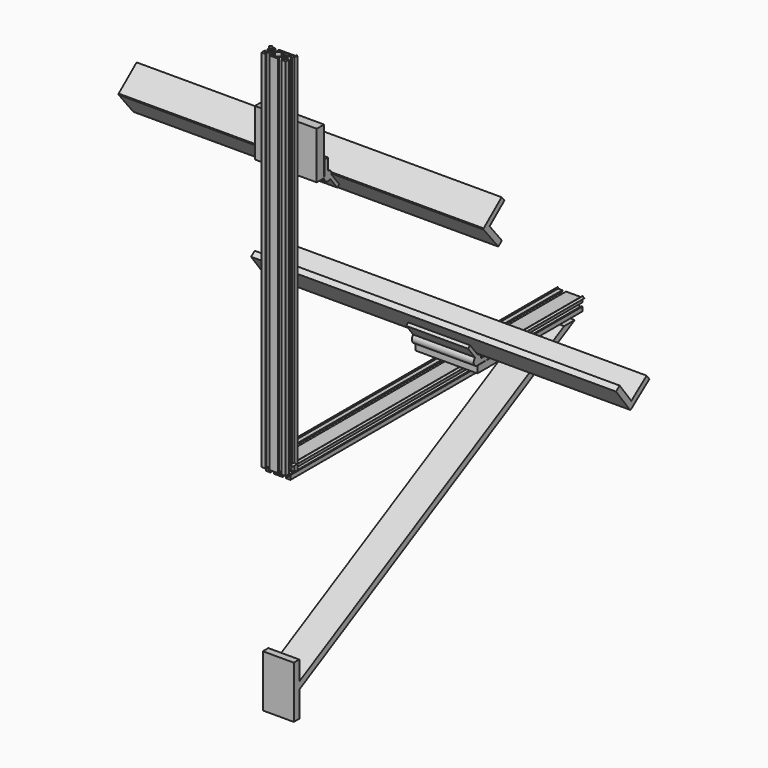
from build123d import *

# Parameters (mm, degrees)
F0_R          = 2.1
F1_DEPTH      = 600
F2_R          = 2.1
F3_DEPTH      = 600
F5_DEPTH      = 25.4
F5_DEPTH_BACK = 25.4
F6_W          = 67.6259994507
F6_H          = 11.4020574838
F7_DEPTH      = 50.8
F7_DEPTH_BACK = 50.8
F6_W_2        = 15.0790625318
F6_H_2        = 77.6842328595
F9_DEPTH      = 300
F9_DEPTH_BACK = 300


with BuildPart() as f1:
    # F0 (on Front) → F1 (new body)
    with BuildSketch(Plane.XZ):
        Polygon((16, -10), (20, -10), (20, -6), (20, -3), (18, -3), (18, -6), (17, -6), (13, -2), (13, 2), (17, 6), (18, 6), (18, 3), (20, 3), (20, 6), (20, 7.62), (20.4436164349, 7.62), (23.18, 10), (20.4436164349, 12.38), (20, 12.38), (20, 10), (16, 10), (-7, 10), (-7, 8), (-3, 8), (-8, 3), (-12, 3), (-16, 7), (-16, 8), (-13, 8), (-13, 10), (-16, 10), (-19, 10), (-20, 10), (-20, 12.38), (-20.4436164349, 12.38), (-23.18, 10), (-20.4436164349, 7.62), (-20, 7.62), (-20, 6), (-20, 3), (-18, 3), (-18, 6), (-17, 6), (-13, 2), (-13, -2), (-17, -6), (-18, -6), (-18, -3), (-20, -3), (-20, -6), (-20, -10), (-16, -10), (-13, -10), (-13, -8), (-16, -8), (-16, -7), (-12, -3), (-8, -3), (-3, -8), (-7, -8), (-7, -10), (-1, -10), (0, -10), (7, -10), (7, -8), (3, -8), (8, -3), (12, -3), (16, -7), (16, -8), (13, -8), (13, -10), align=None)
        with Locations((-10, 0)):
            Circle(F0_R, mode=Mode.SUBTRACT)
        Polygon((-2, -7), (-7, -2), (-7, 2), (-2, 7), (-1, 8), (1, 8), (2, 7), (7, 2), (7, -2), (2, -7), (1, -8), (-1, -8), align=None, mode=Mode.SUBTRACT)
        with Locations((10, 0)):
            Circle(F0_R, mode=Mode.SUBTRACT)
        Polygon((12, 3), (8, 3), (3, 8), (16, 8), (16, 7), align=None, mode=Mode.SUBTRACT)
    extrude(amount=-F1_DEPTH)

    # F2 (on Top) → F3 (join)
    with BuildSketch(Plane.XY):
        Polygon((16.4503816794, -10.3344274809), (20.4503816794, -10.3344274809), (20.4503816794, -6.3344274809), (20.4503816794, -3.3344274809), (18.4503816794, -3.3344274809), (18.4503816794, -6.3344274809), (17.4503816794, -6.3344274809), (13.4503816794, -2.3344274809), (13.4503816794, 1.6655725191), (17.4503816794, 5.6655725191), (18.4503816794, 5.6655725191), (18.4503816794, 2.6655725191), (20.4503816794, 2.6655725191), (20.4503816794, 5.6655725191), (20.4503816794, 7.2855725191), (20.8939981143, 7.2855725191), (23.6303816794, 9.6655725191), (20.8939981143, 12.0455725191), (20.4503816794, 12.0455725191), (20.4503816794, 9.6655725191), (16.4503816794, 9.6655725191), (-6.5496183206, 9.6655725191), (-6.5496183206, 7.6655725191), (-2.5496183206, 7.6655725191), (-7.5496183206, 2.6655725191), (-11.5496183206, 2.6655725191), (-15.5496183206, 6.6655725191), (-15.5496183206, 7.6655725191), (-12.5496183206, 7.6655725191), (-12.5496183206, 9.6655725191), (-15.5496183206, 9.6655725191), (-18.5496183206, 9.6655725191), (-19.5496183206, 9.6655725191), (-19.5496183206, 12.0455725191), (-19.9932347555, 12.0455725191), (-22.7296183206, 9.6655725191), (-19.9932347555, 7.2855725191), (-19.5496183206, 7.2855725191), (-19.5496183206, 5.6655725191), (-19.5496183206, 2.6655725191), (-17.5496183206, 2.6655725191), (-17.5496183206, 5.6655725191), (-16.5496183206, 5.6655725191), (-12.5496183206, 1.6655725191), (-12.5496183206, -2.3344274809), (-16.5496183206, -6.3344274809), (-17.5496183206, -6.3344274809), (-17.5496183206, -3.3344274809), (-19.5496183206, -3.3344274809), (-19.5496183206, -6.3344274809), (-19.5496183206, -10.3344274809), (-15.5496183206, -10.3344274809), (-12.5496183206, -10.3344274809), (-12.5496183206, -8.3344274809), (-15.5496183206, -8.3344274809), (-15.5496183206, -7.3344274809), (-11.5496183206, -3.3344274809), (-7.5496183206, -3.3344274809), (-2.5496183206, -8.3344274809), (-6.5496183206, -8.3344274809), (-6.5496183206, -10.3344274809), (-0.5496183206, -10.3344274809), (0.4503816794, -10.3344274809), (7.4503816794, -10.3344274809), (7.4503816794, -8.3344274809), (3.4503816794, -8.3344274809), (8.4503816794, -3.3344274809), (12.4503816794, -3.3344274809), (16.4503816794, -7.3344274809), (16.4503816794, -8.3344274809), (13.4503816794, -8.3344274809), (13.4503816794, -10.3344274809), align=None)
        with Locations((-9.5496183206, -0.3344274809)):
            Circle(F2_R, mode=Mode.SUBTRACT)
        Polygon((-1.5496183206, -7.3344274809), (-6.5496183206, -2.3344274809), (-6.5496183206, 1.6655725191), (-1.5496183206, 6.6655725191), (-0.5496183206, 7.6655725191), (1.4503816794, 7.6655725191), (2.4503816794, 6.6655725191), (7.4503816794, 1.6655725191), (7.4503816794, -2.3344274809), (2.4503816794, -7.3344274809), (1.4503816794, -8.3344274809), (-0.5496183206, -8.3344274809), align=None, mode=Mode.SUBTRACT)
        with Locations((10.4503816794, -0.3344274809)):
            Circle(F2_R, mode=Mode.SUBTRACT)
        Polygon((12.4503816794, 2.6655725191), (8.4503816794, 2.6655725191), (3.4503816794, 7.6655725191), (16.4503816794, 7.6655725191), (16.4503816794, 6.6655725191), align=None, mode=Mode.SUBTRACT)
    extrude(amount=F3_DEPTH)


with BuildPart() as f5:
    # F4 (on Right) → F5 (new body, two sides)
    with BuildSketch(Plane.YZ) as f5_sk:
        Polygon((577.4232465298, -11.5676193306), (577.0964622498, -11.5676193306), (577.0964622498, -11.7435521713), align=None)
        Polygon((577.0964622498, -11.7435521713), (577.0964622498, -11.5676193306), (555.6103307278, -11.5676193306), (11.2802451476, -304.6219187382), (11.2802451476, -291.0836935043), (11.2802451476, -272.7263271809), (0, -272.7263271809), (0, -291.0836935043), (0, -310.6949329376), (0, -322.4384851089), (0, -358.4799766541), (11.2802451476, -358.4799766541), (11.2802451476, -316.3654709095), align=None)
    extrude(amount=F5_DEPTH)
    extrude(f5_sk.sketch, amount=-F5_DEPTH_BACK)


with BuildPart() as f7:
    # F6 (on Right) → F7 (new body, two sides)
    with BuildSketch(Plane.YZ) as f7_sk:
        with Locations((379.4575035572, 19.3334678188)):
            Rectangle(F6_W, F6_H)
    extrude(amount=F7_DEPTH)
    extrude(f7_sk.sketch, amount=-F7_DEPTH_BACK)


with BuildPart() as f7b:
    # F6 (on Right) → F7, piece 2 (new body, two sides)
    with BuildSketch(Plane.YZ) as f7_2_sk:
        with BuildLine():
            ThreePointArc((340.9104562797, 38.732160941), (338.3981734553, 30.1969923926), (345.6445038319, 25.0344965607))
            ThreePointArc((345.6445038319, 25.0344965607), (346.6697853367, 25.1033604136), (347.676648747, 25.3087149061))
            Line((347.676648747, 25.3087149061), (347.676648747, 32.701395452))
            Line((347.676648747, 32.701395452), (345.6445038319, 32.701395452))
            Line((345.6445038319, 32.701395452), (340.9104562797, 38.732160941))
        make_face()
        with BuildLine():
            Line((347.676648747, 32.701395452), (347.676648747, 25.3087149061))
            ThreePointArc((347.676648747, 25.3087149061), (351.742109436, 28.0537568574), (353.3114027232, 32.701395452))
            Line((353.3114027232, 32.701395452), (347.676648747, 32.701395452))
        make_face()
        with BuildLine():
            ThreePointArc((353.3114027232, 32.701395452), (351.742109436, 28.0537568574), (347.676648747, 25.3087149061))
            Line((347.676648747, 25.3087149061), (374.1813004017, 25.3087149061))
            Line((374.1813004017, 25.3087149061), (374.1813004017, 32.701395452))
            Line((374.1813004017, 32.701395452), (353.3114027232, 32.701395452))
        make_face()
        with BuildLine():
            Line((326.322950049, 57.3153771373), (340.9104562797, 38.732160941))
            ThreePointArc((340.9104562797, 38.732160941), (343.5315072845, 40.0713740274), (346.4639791391, 40.3243737959))
            Line((346.4639791391, 40.3243737959), (330.5324480624, 60.6197609345))
            Line((330.5324480624, 60.6197609345), (326.322950049, 57.3153771373))
        make_face()
        with BuildLine():
            ThreePointArc((346.4639791391, 40.3243737959), (343.5315072845, 40.0713740274), (340.9104562797, 38.732160941))
            Line((340.9104562797, 38.732160941), (345.6445038319, 32.701395452))
            Line((345.6445038319, 32.701395452), (347.676648747, 32.701395452))
            Line((347.676648747, 32.701395452), (353.3114027232, 32.701395452))
            ThreePointArc((353.3114027232, 32.701395452), (351.3481944325, 37.8247978511), (346.4639791391, 40.3243737959))
        make_face()
    extrude(amount=F7_DEPTH)
    extrude(f7_2_sk.sketch, amount=-F7_DEPTH_BACK)


with BuildPart() as f7c:
    # F6 (on Right) → F7, piece 3 (new body, two sides)
    with BuildSketch(Plane.YZ) as f7_3_sk:
        with BuildLine():
            Line((38.2286199435, 426.7386130083), (38.2286199435, 424.3225363208))
            Line((38.2286199435, 424.3225363208), (42.9626674957, 418.2917708318))
            ThreePointArc((42.9626674957, 418.2917708318), (44.8859979515, 420.5198193095), (45.8281406629, 423.3083255713))
            ThreePointArc((45.8281406629, 423.3083255713), (45.878655747, 423.8143131261), (45.8955188348, 424.3225363208))
            ThreePointArc((45.8955188348, 424.3225363208), (43.6499361402, 429.7438525176), (38.2286199435, 431.9894352122))
            Line((38.2286199435, 431.9894352122), (38.2286199435, 426.7386130083))
        make_face()
        with BuildLine():
            Line((42.9626674957, 418.2917708318), (38.2286199435, 424.3225363208))
            Line((38.2286199435, 424.3225363208), (38.2286199435, 426.7386130083))
            Line((38.2286199435, 426.7386130083), (30.9523632101, 426.7386130083))
            ThreePointArc((30.9523632101, 426.7386130083), (30.6600116404, 425.5462629912), (30.5617210522, 424.3225363208))
            ThreePointArc((30.5617210522, 424.3225363208), (34.8755709817, 417.4277265867), (42.9626674957, 418.2917708318))
        make_face()
        with BuildLine():
            ThreePointArc((45.8281406629, 423.3083255713), (44.8859979515, 420.5198193095), (42.9626674957, 418.2917708318))
            Line((42.9626674957, 418.2917708318), (57.5501737264, 399.7085546355))
            Line((57.5501737264, 399.7085546355), (61.7596717397, 403.0129384327))
            Line((61.7596717397, 403.0129384327), (45.8281406629, 423.3083255713))
        make_face()
        with BuildLine():
            Line((30.9523632101, 426.7386130083), (38.2286199435, 426.7386130083))
            Line((38.2286199435, 426.7386130083), (38.2286199435, 431.9894352122))
            ThreePointArc((38.2286199435, 431.9894352122), (33.7421111152, 430.5396560031), (30.9523632101, 426.7386130083))
        make_face()
        with BuildLine():
            ThreePointArc((30.9523632101, 426.7386130083), (33.7421111152, 430.5396560031), (38.2286199435, 431.9894352122))
            Line((38.2286199435, 431.9894352122), (38.2286199435, 451.1919021606))
            Line((38.2286199435, 451.1919021606), (30.9523632101, 451.1919021606))
            Line((30.9523632101, 451.1919021606), (30.9523632101, 426.7386130083))
        make_face()
    extrude(amount=F7_DEPTH)
    extrude(f7_3_sk.sketch, amount=-F7_DEPTH_BACK)


with BuildPart() as f7d:
    # F6 (on Right) → F7, piece 4 (new body, two sides)
    with BuildSketch(Plane.YZ) as f7_4_sk:
        with Locations((23.0221897863, 463.1646527506)):
            Rectangle(F6_W_2, F6_H_2)
    extrude(amount=F7_DEPTH)
    extrude(f7_4_sk.sketch, amount=-F7_DEPTH_BACK)


with BuildPart() as f9:
    # F8 (on Right) → F9 (new body, two sides)
    with BuildSketch(Plane.YZ) as f9_sk:
        Polygon((46.9310618937, 426.0134952692), (46.9310618937, 424.1959154606), (77.1296024323, 387.3319327831), (84.4074771326, 393.2938820412), (59.1799772639, 424.0896126151), (89.6657304769, 449.0631826796), (83.8036795212, 456.2191094571), align=None)
    extrude(amount=F9_DEPTH)
    extrude(f9_sk.sketch, amount=-F9_DEPTH_BACK)


with BuildPart() as f9b:
    # F8 (on Right) → F9, piece 2 (new body, two sides)
    with BuildSketch(Plane.YZ) as f9_2_sk:
        Polygon((347.5880919454, 41.1849674582), (349.3536787328, 40.7533430187), (387.4514590367, 69.3982063469), (381.8923054501, 76.7919023681), (350.3936052483, 53.1087388058), (326.4696326599, 84.9277159546), (318.9499367649, 79.2738258995), align=None)
    extrude(amount=F9_DEPTH)
    extrude(f9_2_sk.sketch, amount=-F9_DEPTH_BACK)


solid = Compound([f1.part, f5.part, f7.part, f7b.part, f7c.part, f7d.part, f9.part, f9b.part])
